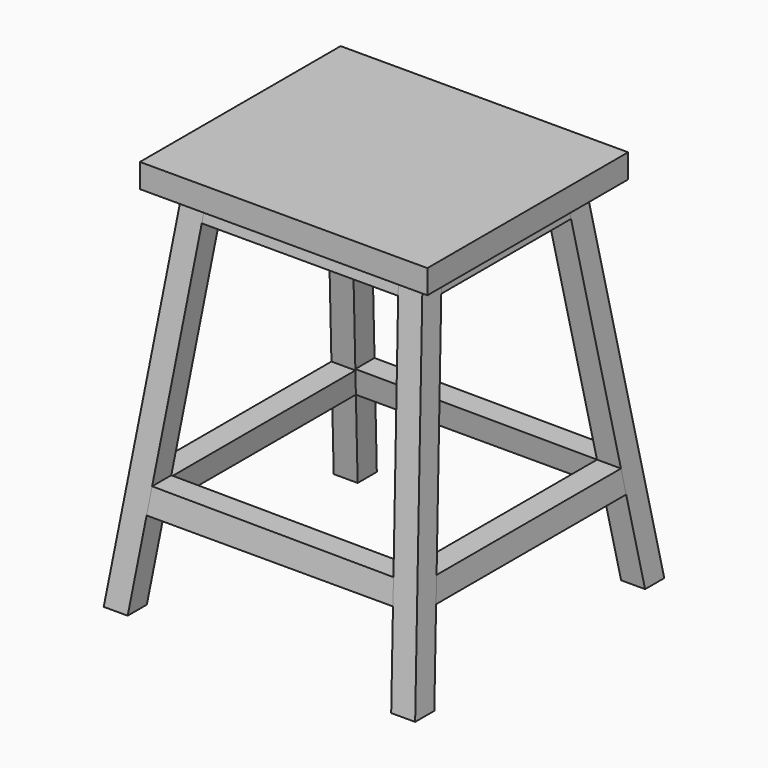
from build123d import *

# Parameters (mm, degrees)
F0_W     = 60
F0_H     = 52.3636344809
F1_DEPTH = 5
F2_W     = 5
F2_H     = 5
F4_W     = 5
F4_H     = 5


with BuildPart() as f1:
    # F0 (on Top) → F1 (new body)
    with BuildSketch(Plane.XY):
        Rectangle(F0_W, F0_H)
    extrude(amount=F1_DEPTH)



with BuildPart() as f5:
    # F2 (on Top) → F5 section 0
    with BuildSketch(Plane.XY):
        with Locations((-22.5, -18.6818172405)):
            Rectangle(F2_W, F2_H)
    # F4 (on offset) → F5 section 1
    with BuildSketch(Plane.XY.offset(-75)):
        with Locations((-30, -30)):
            Rectangle(F4_W, F4_H)
    loft()


with BuildPart() as f6_1:
    # F6: instance of F5
    add(f5.part.mirror(Plane.YZ))


with BuildPart() as f1_1:
    add(f1.part)

    add(f5.part)  # F7 merges F5

    add(f6_1.part)  # F7 merges F6_1
    # F7: F5, F6_1 across plane
    add(f5.part.mirror(Plane.XZ))
    add(f6_1.part.mirror(Plane.XZ))



with BuildPart() as f10:
    # F9 (on face) → F10 section 0
    with BuildSketch(Plane(origin=(-19.801980198, 0, 1.9801980198), x_dir=(0, 1, 0), z_dir=(0.9950371902, 0, -0.099503719))):
        Polygon((21.1818172405, -1.9900743804), (16.1818172405, -1.9900743804), (16.9242940412, -6.9346399023), (21.9242940412, -6.9346399023), align=None)
    # F8 (on face) → F10 section 1
    with BuildSketch(Plane(origin=(19.801980198, 0, 1.9801980198), x_dir=(0, -1, 0), z_dir=(-0.9950371902, 0, -0.099503719))):
        Polygon((-16.1818172405, -1.9900743804), (-21.1818172405, -1.9900743804), (-21.9242940412, -6.9346399023), (-16.9242940412, -6.9346399023), align=None)
    loft()


with BuildPart() as f11_1:
    # F11: instance of F10
    add(f10.part.mirror(Plane.XZ))


with BuildPart() as f14:
    # F13 (on face) → F14 section 0
    with BuildSketch(Plane(origin=(0, -15.8215052801, 2.3876091772), x_dir=(-1, 0, 0), z_dir=(0, 0.9888040904, -0.1492195388))):
        Polygon((-20, -2.4146433053), (-25, -2.4146433053), (-25.4944020452, -7.4146433053), (-20.4944020452, -7.4146433053), align=None)
    # F12 (on face) → F14 section 1
    with BuildSketch(Plane(origin=(0, 15.8215052801, 2.3876091772), x_dir=(1, 0, 0), z_dir=(0, -0.9888040904, -0.1492195388))):
        Polygon((25, -2.4146433053), (20, -2.4146433053), (20.4944020452, -7.4146433053), (25.4944020452, -7.4146433053), align=None)
    loft()


with BuildPart() as f1_2:
    add(f1_1.part)

    add(f10.part)  # F15 merges F10

    add(f11_1.part)  # F15 merges F11_1

    add(f14.part)  # F15 merges F14
    # F15: F14 across plane
    add(f14.part.mirror(Plane.YZ))



with BuildPart() as f18:
    # F17 (on face) → F18 section 0
    with BuildSketch(Plane(origin=(19.801980198, 0, 1.9801980198), x_dir=(0, -1, 0), z_dir=(-0.9950371902, 0, -0.099503719))):
        Polygon((-29.7971169349, -59.3641415388), (-24.7971169349, -59.3641415388), (-24.0546401341, -54.4195760169), (-29.0546401341, -54.4195760169), align=None)
    # F16 (on face) → F18 section 1
    with BuildSketch(Plane(origin=(-19.801980198, 0, 1.9801980198), x_dir=(0, 1, 0), z_dir=(0.9950371902, 0, -0.099503719))):
        Polygon((29.0120788259, -54.1361366195), (24.0120788259, -54.1361366195), (24.7971169349, -59.3641415388), (29.7971169349, -59.3641415388), align=None)
    loft()


with BuildPart() as f1_3:
    add(f1_2.part)

    add(f18.part)  # F19 merges F18
    # F19: F18 across plane
    add(f18.part.mirror(Plane.XZ))



with BuildPart() as f22:
    # F21 (on face) → F22 section 0
    with BuildSketch(Plane(origin=(0, -15.8215052801, 2.3876091772), x_dir=(-1, 0, 0), z_dir=(0, 0.9888040904, -0.1492195388))):
        Polygon((-30.7089330576, -60.1503779457), (-25.7089330576, -60.1503779457), (-25.2169303993, -55.174643489), (-30.2169303993, -55.174643489), align=None)
    # F20 (on face) → F22 section 1
    with BuildSketch(Plane(origin=(0, 15.8215052801, 2.3876091772), x_dir=(1, 0, 0), z_dir=(0, -0.9888040904, -0.1492195388))):
        Polygon((30.2169303993, -55.174643489), (25.2169303993, -55.174643489), (25.7089330576, -60.1503779457), (30.7089330576, -60.1503779457), align=None)
    loft()


with BuildPart() as f1_4:
    add(f1_3.part)

    add(f22.part)  # F23 merges F22
    # F23: F22 across plane
    add(f22.part.mirror(Plane.YZ))


solid = f1_4.part
